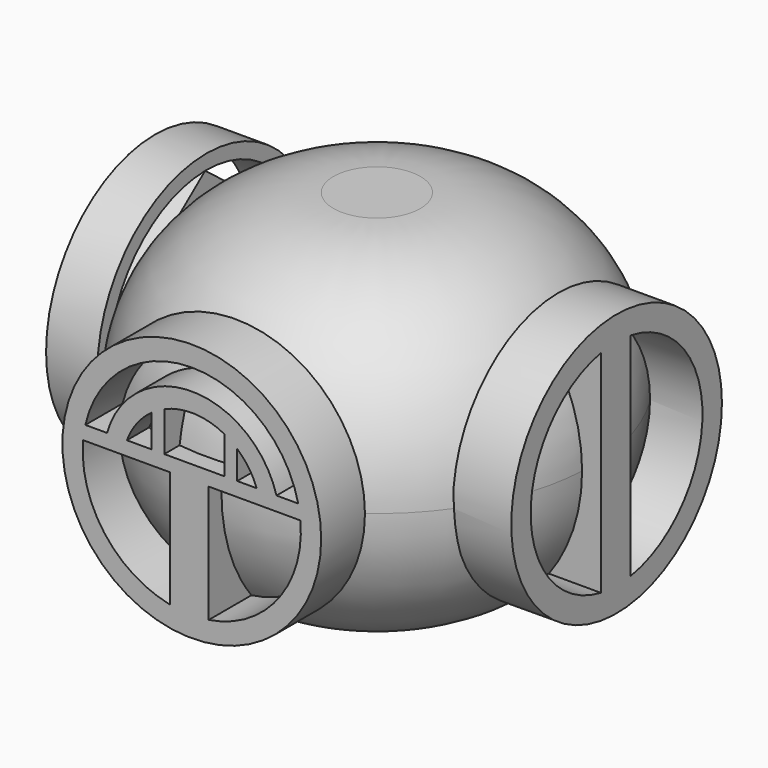
from build123d import *

# Parameters (mm, degrees)
F0_R      = 15.9252412
F1_DEPTH  = 25.4
F2_R      = 12.69999
F4_R      = 9.6084759936
F5_DEPTH  = 4.064
F7_R      = 9.7784172286
F8_DEPTH  = 4.318
F10_R     = 10.1162492157
F10_W     = 5.6749439845
F10_H     = 1.978664659
F10_H_2   = 1.6942825168
F11_DEPTH = 3.81


# Not quite as in the source:
# - a fillet or chamfer is up to 0.001 mm smaller than in the source, because OpenCascade refuses the exact size


with BuildPart() as f1:
    # F0 (on Top) → F1 (new body)
    with BuildSketch(Plane.XY):
        with Locations((-32.790163897, 15.5415115881)):
            Circle(F0_R)
    extrude(amount=F1_DEPTH)

    # F2 (radius 12.7 in the source; OpenCascade refuses exactly that, so slightly less here)
    f2_edges = [f1.edges().sort_by_distance(p)[0] for p in [
        (-48.715405, 15.541512, 25.4),
        (-48.715405, 15.541512, 0),
    ]]
    fillet(f2_edges, radius=F2_R)

    # F4 (on offset) → F5 (join)
    with BuildSketch(Plane.XZ.offset(-2.54)):
        with Locations((-32.8846593334, 12.7722686057)):
            Circle(F4_R)
        with BuildLine():
            ThreePointArc((-34.4953425229, 4.8360576775), (-39.3760068955, 7.9307656301), (-40.9506916141, 13.4912035685))
            Line((-40.9506916141, 13.4912035685), (-34.4953425229, 13.4912035685))
            Line((-34.4953425229, 13.4912035685), (-34.4953425229, 4.8360576775))
        make_face(mode=Mode.SUBTRACT)
        with BuildLine():
            Line((-31.6289104521, 4.8360576775), (-31.6289104521, 13.4912035685))
            Line((-31.6289104521, 13.4912035685), (-24.8186270527, 13.4912035685))
            ThreePointArc((-24.8186270527, 13.4912035685), (-26.5027249618, 7.7874257887), (-31.6289104521, 4.7722161695))
            Line((-31.6289104521, 4.7722161695), (-31.6289104521, 4.8360576775))
        make_face(mode=Mode.SUBTRACT)
        with BuildLine():
            Line((-35.8861955936, 14.5410663136), (-37.7050013264, 14.5410663136))
            ThreePointArc((-37.7050013264, 14.5410663136), (-36.9751394, 15.875865726), (-35.8861955936, 16.9382165577))
            Line((-35.8861955936, 16.9382165577), (-35.8861955936, 14.5410663136))
        make_face(mode=Mode.SUBTRACT)
        with BuildLine():
            Line((-34.9271344844, 14.5410663136), (-34.9271344844, 17.4831748368))
            ThreePointArc((-34.9271344844, 17.4831748368), (-32.671720338, 17.9024732063), (-30.4588118953, 17.2977085255))
            Line((-30.4588118953, 17.2977085255), (-30.4588118953, 14.5410663136))
            Line((-30.4588118953, 14.5410663136), (-34.9271344844, 14.5410663136))
        make_face(mode=Mode.SUBTRACT)
        with BuildLine():
            ThreePointArc((-29.5103743217, 16.6424808634), (-28.654770007, 15.6830036583), (-28.0643173404, 14.5410663136))
            Line((-28.0643173404, 14.5410663136), (-29.5103743217, 14.5410663136))
            Line((-29.5103743217, 14.5410663136), (-29.5103743217, 16.6424808634))
        make_face(mode=Mode.SUBTRACT)
        with BuildLine():
            ThreePointArc((-40.78713356, 14.5410663136), (-32.8846593334, 20.8702772642), (-24.9821851068, 14.5410663136))
            Line((-24.9821851068, 14.5410663136), (-26.5939201863, 14.5410663136))
            ThreePointArc((-26.5939201863, 14.5410663136), (-32.8846593334, 19.3069487316), (-39.1753984805, 14.5410663136))
            Line((-39.1753984805, 14.5410663136), (-40.78713356, 14.5410663136))
        make_face(mode=Mode.SUBTRACT)
    extrude(amount=F5_DEPTH)

    # F7 (on offset) → F8 (join)
    with BuildSketch(Plane.YZ.offset(-19.812)):
        with Locations((16.1675531426, 13.0318262674)):
            Circle(F7_R)
        with BuildLine():
            ThreePointArc((14.7082107462, 5.1923968714), (8.1934492128, 13.0318262674), (14.7082107462, 20.8712556633))
            Line((14.7082107462, 20.8712556633), (14.7082107462, 5.1923968714))
        make_face(mode=Mode.SUBTRACT)
        with BuildLine():
            Line((17.472269508, 5.1651847547), (17.472269508, 20.89846778))
            ThreePointArc((17.472269508, 20.89846778), (24.1416570724, 13.0318262674), (17.472269508, 5.1651847547))
        make_face(mode=Mode.SUBTRACT)
    extrude(amount=F8_DEPTH)

    # F10 (on offset) → F11 (join)
    with BuildSketch(Plane.YZ.offset(-45.974)):
        with Locations((16.1922425032, 13.2868457586)):
            Circle(F10_R)
        with BuildLine():
            ThreePointArc((18.5630126357, 4.5764919974), (14.1502134499, 4.4936136445), (10.2255434294, 6.5126804351))
            Line((10.2255434294, 6.5126804351), (14.5346437458, 9.6941854786))
            Line((14.5346437458, 9.6941854786), (18.5630126357, 4.5764919974))
        make_face(mode=Mode.SUBTRACT)
        with BuildLine():
            Line((7.1966450097, 14.0418552967), (9.6143750356, 15.9449603685))
            Line((9.6143750356, 15.9449603685), (14.1980923483, 10.1217448556))
            Line((14.1980923483, 10.1217448556), (9.8219484974, 6.8907400726))
            ThreePointArc((9.8219484974, 6.8907400726), (7.7180305853, 10.1758095907), (7.1966450097, 14.0418552967))
        make_face(mode=Mode.SUBTRACT)
        Polygon((14.7251297148, 10.5108683191), (12.8217059723, 12.9290031884), (18.0003046989, 12.9290031884), align=None, mode=Mode.SUBTRACT)
        Polygon((18.9159519085, 12.9290031884), (18.9159519085, 5.1867919974), (15.0616811123, 10.0833089421), align=None, mode=Mode.SUBTRACT)
        with BuildLine():
            Line((19.7446108451, 4.9879607232), (19.7446108451, 18.2193573564))
            Line((19.7446108451, 18.2193573564), (25.187377814, 14.0473419168))
            ThreePointArc((25.187377814, 14.0473419168), (23.9303339268, 8.6378937492), (19.7446108451, 4.9879607232))
        make_face(mode=Mode.SUBTRACT)
        Polygon((10.1289065252, 16.3499714645), (12.5037992559, 18.2193573564), (12.5037992559, 13.3328761143), align=None, mode=Mode.SUBTRACT)
        with Locations((16.0784799163, 14.6003742702)):
            Rectangle(F10_W, F10_H, mode=Mode.SUBTRACT)
        with Locations((16.0784799163, 17.372216098)):
            Rectangle(F10_W, F10_H_2, mode=Mode.SUBTRACT)
        with BuildLine():
            ThreePointArc((7.445538155, 15.5197758319), (10.605122595, 20.3773256293), (16.0669122977, 22.3132019451))
            Line((16.0669122977, 22.3132019451), (16.0755219814, 22.3128279156))
            Line((16.0755219814, 22.3128279156), (7.445538155, 15.5197758319))
        make_face(mode=Mode.SUBTRACT)
        Polygon((13.3107499921, 18.8545449177), (15.7857291495, 20.8027133801), (15.7857291495, 18.8545449177), align=None, mode=Mode.SUBTRACT)
        Polygon((16.3304693817, 20.8363811937), (18.9159519085, 18.8545449177), (16.3304693817, 18.8545449177), align=None, mode=Mode.SUBTRACT)
        with BuildLine():
            ThreePointArc((16.0840874609, 22.3134240778), (21.687199068, 20.44898692), (24.9389468513, 15.5197758319))
            Line((24.9389468513, 15.5197758319), (16.0768654888, 22.3127802877))
            Line((16.0768654888, 22.3127802877), (16.0840874609, 22.3134240778))
        make_face(mode=Mode.SUBTRACT)
    extrude(amount=-F11_DEPTH)


solid = f1.part
